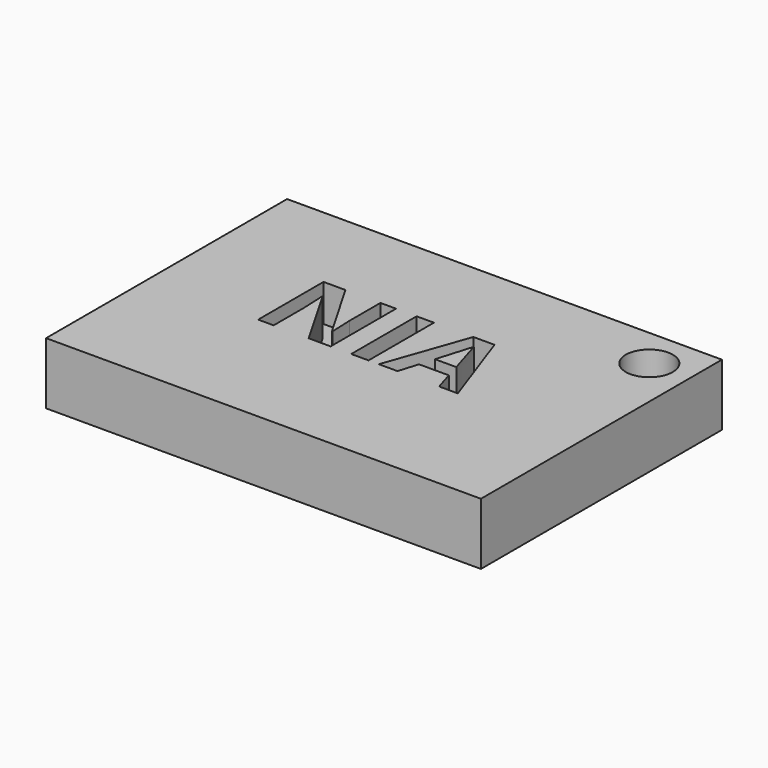
from build123d import *

# Parameters (mm, degrees)
F0_W         = 44.6771159768
F0_H         = 30.9527758509
F1_DEPTH     = 6.35
F4_D         = 4.826
F2_TEXT_SIZE = 11.7614050396
F5_DEPTH     = 3.81


# Not quite as in the source:
# - Text() gives the source's letters only with a copy of the font that has no kerning and outlines rounded to 1/6400 em; it was checked with that copy


with BuildPart() as f1:
    # F0 (on Top) → F1 (new body)
    with BuildSketch(Plane.XY):
        with Locations((-22.3385579884, 15.4763879254)):
            Rectangle(F0_W, F0_H)
    extrude(amount=F1_DEPTH)

    # F4 (through all)
    with Locations(Plane.XY.offset(6.35)):
        with Locations((-4.1464077282, 26.8122157934)):
            Hole(F4_D / 2)

    # F2 (on face) → F5 (cut)
    with BuildSketch(Plane.XY.offset(6.35)):
        with Locations((-34.4568621367, 13.1403291598)):
            Text('NIA', F2_TEXT_SIZE, font='Open Sans', font_style=FontStyle.BOLD, text_align=(TextAlign.LEFT, TextAlign.BOTTOM))
    extrude(amount=-F5_DEPTH, mode=Mode.SUBTRACT)


solid = f1.part
